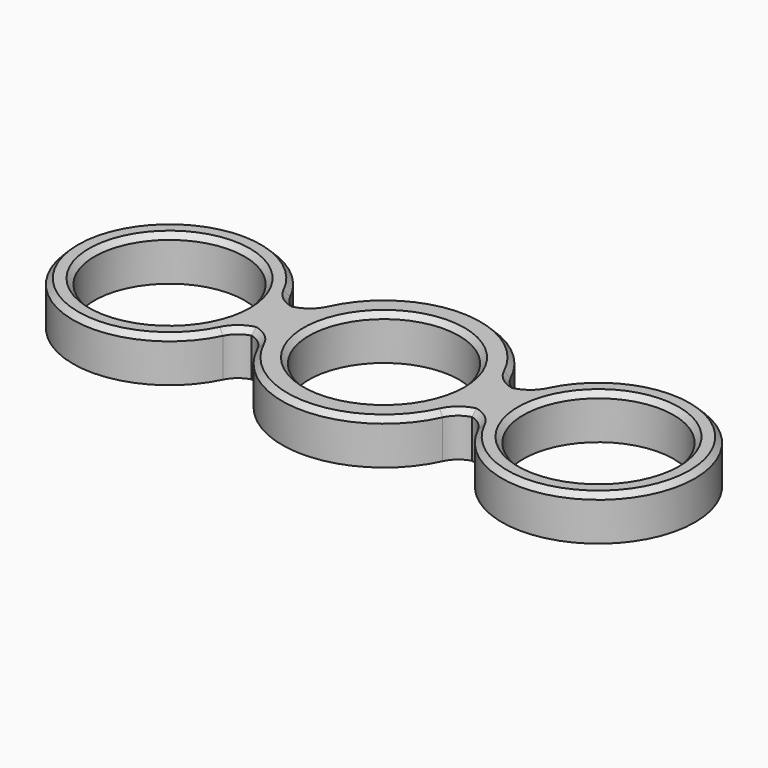
from build123d import *

# Parameters (mm, degrees)
F0_R        = 14.01
F1_DEPTH    = 8.2
F2_T1_DEPTH = 8.2
F3_C1_SIZE  = 1
F3_C2_SIZE  = 1
F3_C3_SIZE  = 1
F3_C4_SIZE  = 1
F3_C5_SIZE  = 1
F3_C6_SIZE  = 1
F3_C7_SIZE  = 1


# Not quite as in the source:
# - a fillet or chamfer that OpenCascade refuses, or shapes differently, is made with other operations: its cross-section is extruded or revolved along the edge and cut away or added


with BuildPart() as f1:
    # F0 (on Top) → F1 (new body)
    with BuildSketch(Plane.XY):
        with BuildLine():
            Line((-22.6979741071, -5), (-18.3303027798, -5))
            ThreePointArc((-18.3303027798, -5), (0, -19), (18.3303027798, -5))
            Line((18.3303027798, -5), (22.6979741071, -5))
            ThreePointArc((22.6979741071, -5), (58.01, 0), (22.6979741071, 5))
            Line((22.6979741071, 5), (18.3303027798, 5))
            ThreePointArc((18.3303027798, 5), (0, 19), (-18.3303027798, 5))
            Line((-18.3303027798, 5), (-22.6979741071, 5))
            ThreePointArc((-22.6979741071, 5), (-58.01, 0), (-22.6979741071, -5))
        make_face()
        with Locations((-40, 0)):
            Circle(F0_R, mode=Mode.SUBTRACT)
        Circle(F0_R, mode=Mode.SUBTRACT)
        with Locations((40, 0)):
            Circle(F0_R, mode=Mode.SUBTRACT)
    extrude(amount=F1_DEPTH)

    # F2: fillet of radius 5 on 8 edges, made by hand

    # F2_s2 → F2_t1 (join)
    with BuildSketch(Plane.XY):
        with BuildLine():
            ThreePointArc((-19.2765808806, -5), (-21.9350728052, -5.7653311007), (-23.7797141095, -7.8270317253))
            ThreePointArc((-23.7797141095, -7.8270317253), (-23.1793468046, -6.4362820074), (-22.6979741071, -5))
            Line((-22.6979741071, -5), (-19.2765808806, -5))
        make_face()
        with BuildLine():
            ThreePointArc((-21.8174242293, -5), (-19.1171156049, -5.7918729423), (-17.2721275148, -7.9166666667))
            ThreePointArc((-17.2721275148, -7.9166666667), (-17.8608509549, -6.4799693801), (-18.3303027798, -5))
            Line((-18.3303027798, -5), (-21.8174242293, -5))
        make_face()
        with BuildLine():
            ThreePointArc((17.2721275148, -7.9166666667), (19.1171156049, -5.7918729423), (21.8174242293, -5))
            Line((21.8174242293, -5), (18.3303027798, -5))
            ThreePointArc((18.3303027798, -5), (17.8608509549, -6.4799693801), (17.2721275148, -7.9166666667))
        make_face()
        with BuildLine():
            ThreePointArc((19.2765808806, -5), (21.9350728052, -5.7653311007), (23.7797141095, -7.8270317253))
            ThreePointArc((23.7797141095, -7.8270317253), (23.1793468046, -6.4362820074), (22.6979741071, -5))
            Line((22.6979741071, -5), (19.2765808806, -5))
        make_face()
        with BuildLine():
            ThreePointArc((21.8174242293, 5), (19.1171156049, 5.7918729423), (17.2721275148, 7.9166666667))
            ThreePointArc((17.2721275148, 7.9166666667), (17.8608509549, 6.4799693801), (18.3303027798, 5))
            Line((18.3303027798, 5), (21.8174242293, 5))
        make_face()
        with BuildLine():
            ThreePointArc((23.7797141095, 7.8270317253), (21.9350728052, 5.7653311007), (19.2765808806, 5))
            Line((19.2765808806, 5), (22.6979741071, 5))
            ThreePointArc((22.6979741071, 5), (23.1793468046, 6.4362820074), (23.7797141095, 7.8270317253))
        make_face()
        with BuildLine():
            ThreePointArc((-17.2721275148, 7.9166666667), (-19.1171156049, 5.7918729423), (-21.8174242293, 5))
            Line((-21.8174242293, 5), (-18.3303027798, 5))
            ThreePointArc((-18.3303027798, 5), (-17.8608509549, 6.4799693801), (-17.2721275148, 7.9166666667))
        make_face()
        with BuildLine():
            ThreePointArc((-19.2765808806, 5), (-21.9350728052, 5.7653311007), (-23.7797141095, 7.8270317253))
            ThreePointArc((-23.7797141095, 7.8270317253), (-23.1793468046, 6.4362820074), (-22.6979741071, 5))
            Line((-22.6979741071, 5), (-19.2765808806, 5))
        make_face()
    extrude(amount=F2_T1_DEPTH)

    # F3: chamfer of 1 on 15 edges, made by hand

    # F3_c1
    f3_c1_edges = [f1.edges().sort_by_distance(p)[0] for p in [
        (0, -19, 8.2),
        (18.6003113726, -6.1724440085, 8.2),
        (-18.6003113726, -6.1724440085, 8.2),
    ]]
    chamfer(f3_c1_edges, length=F3_C1_SIZE)

    # F3_c2
    f3_c2_edges = [f1.edges().sort_by_distance(p)[0] for p in [
        (22.4556214842, -6.1407642155, 8.2),
        (58.01, 0, 8.2),
        (22.4556214842, 6.1407642155, 8.2),
    ]]
    chamfer(f3_c2_edges, length=F3_C2_SIZE)

    # F3_c3
    f3_c3_edges = [f1.edges().sort_by_distance(p)[0] for p in [
        (18.6003113726, 6.1724440085, 8.2),
        (0, 19, 8.2),
        (-18.6003113726, 6.1724440085, 8.2),
    ]]
    chamfer(f3_c3_edges, length=F3_C3_SIZE)

    # F3_c4
    f3_c4_edges = [f1.edges().sort_by_distance(p)[0] for p in [
        (-22.4556214842, 6.1407642155, 8.2),
        (-58.01, 0, 8.2),
        (-22.4556214842, -6.1407642155, 8.2),
    ]]
    chamfer(f3_c4_edges, length=F3_C4_SIZE)

    # F3_c5
    f3_c5_edges = [f1.edges().sort_by_distance(p)[0] for p in [
        (-54.01, 0, 8.2),
    ]]
    chamfer(f3_c5_edges, length=F3_C5_SIZE)

    # F3_c6
    f3_c6_edges = [f1.edges().sort_by_distance(p)[0] for p in [
        (-14.01, 0, 8.2),
    ]]
    chamfer(f3_c6_edges, length=F3_C6_SIZE)

    # F3_c7
    f3_c7_edges = [f1.edges().sort_by_distance(p)[0] for p in [
        (25.99, 0, 8.2),
    ]]
    chamfer(f3_c7_edges, length=F3_C7_SIZE)


solid = f1.part
